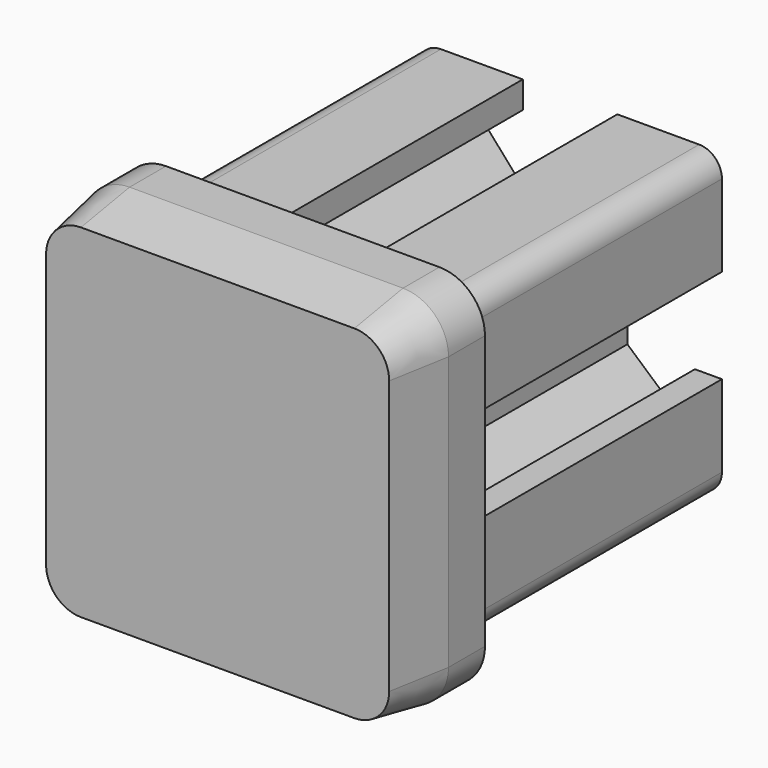
from build123d import *

# Parameters (mm, degrees)
F1_DEPTH = 25
F2_R     = 1.5
F4_DEPTH = 4
F4_TAPER = 10
F5_DEPTH = 3


with BuildPart() as f1:
    # F0 (on Front) → F1 (new body)
    with BuildSketch(Plane.XZ):
        Polygon((10, 3.1115), (10, 10), (3.1115, 10), (3.1115, 8.222), (5.461, 8.222), (5.461, 6.444), (3.1115, 3.777), (0, 3.777), (-3.1115, 3.777), (-5.461, 6.444), (-5.461, 8.222), (-3.1115, 8.222), (-3.1115, 10), (-10, 10), (-10, 3.1115), (-8.222, 3.1115), (-8.222, 5.461), (-6.444, 5.461), (-3.777, 3.1115), (-3.777, 0), (-3.777, -3.1115), (-6.444, -5.461), (-8.222, -5.461), (-8.222, -3.1115), (-10, -3.1115), (-10, -10), (-3.1115, -10), (-3.1115, -8.222), (-5.461, -8.222), (-5.461, -6.444), (-3.1115, -3.777), (0, -3.777), (3.1115, -3.777), (5.461, -6.444), (5.461, -8.222), (3.1115, -8.222), (3.1115, -10), (10, -10), (10, -3.1115), (8.222, -3.1115), (8.222, -5.461), (6.444, -5.461), (3.777, -3.1115), (3.777, 0), (3.777, 3.1115), (6.444, 5.461), (8.222, 5.461), (8.222, 3.1115), align=None)
    extrude(amount=F1_DEPTH)

    # F2
    f2_edges = [f1.edges().sort_by_distance(p)[0] for p in [
        (-10, -12.5, 10),
        (10, -12.5, 10),
        (10, -12.5, -10),
        (-10, -12.5, -10),
    ]]
    fillet(f2_edges, radius=F2_R)


with BuildPart() as f4:
    # F3 (on face) → F4 (new body)
    with BuildSketch(Plane.XZ.offset(25)):
        with BuildLine():
            Line((9, 12), (-9, 12))
            ThreePointArc((-9, 12), (-11.1213203436, 11.1213203436), (-12, 9))
            Line((-12, 9), (-12, -9))
            ThreePointArc((-12, -9), (-11.1213203436, -11.1213203436), (-9, -12))
            Line((-9, -12), (9, -12))
            ThreePointArc((9, -12), (11.1213203436, -11.1213203436), (12, -9))
            Line((12, -9), (12, 9))
            ThreePointArc((12, 9), (11.1213203436, 11.1213203436), (9, 12))
        make_face()
        with BuildLine():
            Line((10, 8.5), (10, 3.1115))
            Line((10, 3.1115), (8.222, 3.1115))
            Line((8.222, 3.1115), (8.222, 5.461))
            Line((8.222, 5.461), (6.444, 5.461))
            Line((6.444, 5.461), (3.777, 3.1115))
            Line((3.777, 3.1115), (3.777, -3.1115))
            Line((3.777, -3.1115), (6.444, -5.461))
            Line((6.444, -5.461), (8.222, -5.461))
            Line((8.222, -5.461), (8.222, -3.1115))
            Line((8.222, -3.1115), (10, -3.1115))
            Line((10, -3.1115), (10, -8.5))
            ThreePointArc((10, -8.5), (9.5606601718, -9.5606601718), (8.5, -10))
            Line((8.5, -10), (3.1115, -10))
            Line((3.1115, -10), (3.1115, -8.222))
            Line((3.1115, -8.222), (5.461, -8.222))
            Line((5.461, -8.222), (5.461, -6.444))
            Line((5.461, -6.444), (3.1115, -3.777))
            Line((3.1115, -3.777), (-3.1115, -3.777))
            Line((-3.1115, -3.777), (-5.461, -6.444))
            Line((-5.461, -6.444), (-5.461, -8.222))
            Line((-5.461, -8.222), (-3.1115, -8.222))
            Line((-3.1115, -8.222), (-3.1115, -10))
            Line((-3.1115, -10), (-8.5, -10))
            ThreePointArc((-8.5, -10), (-9.5606601718, -9.5606601718), (-10, -8.5))
            Line((-10, -8.5), (-10, -3.1115))
            Line((-10, -3.1115), (-8.222, -3.1115))
            Line((-8.222, -3.1115), (-8.222, -5.461))
            Line((-8.222, -5.461), (-6.444, -5.461))
            Line((-6.444, -5.461), (-3.777, -3.1115))
            Line((-3.777, -3.1115), (-3.777, 3.1115))
            Line((-3.777, 3.1115), (-6.444, 5.461))
            Line((-6.444, 5.461), (-8.222, 5.461))
            Line((-8.222, 5.461), (-8.222, 3.1115))
            Line((-8.222, 3.1115), (-10, 3.1115))
            Line((-10, 3.1115), (-10, 8.5))
            ThreePointArc((-10, 8.5), (-9.5606601718, 9.5606601718), (-8.5, 10))
            Line((-8.5, 10), (-3.1115, 10))
            Line((-3.1115, 10), (-3.1115, 8.222))
            Line((-3.1115, 8.222), (-5.461, 8.222))
            Line((-5.461, 8.222), (-5.461, 6.444))
            Line((-5.461, 6.444), (-3.1115, 3.777))
            Line((-3.1115, 3.777), (3.1115, 3.777))
            Line((3.1115, 3.777), (5.461, 6.444))
            Line((5.461, 6.444), (5.461, 8.222))
            Line((5.461, 8.222), (3.1115, 8.222))
            Line((3.1115, 8.222), (3.1115, 10))
            Line((3.1115, 10), (8.5, 10))
            ThreePointArc((8.5, 10), (9.5606601718, 9.5606601718), (10, 8.5))
        make_face(mode=Mode.SUBTRACT)
        with BuildLine():
            Line((8.222, 3.1115), (10, 3.1115))
            Line((10, 3.1115), (10, 8.5))
            ThreePointArc((10, 8.5), (9.5606601718, 9.5606601718), (8.5, 10))
            Line((8.5, 10), (3.1115, 10))
            Line((3.1115, 10), (3.1115, 8.222))
            Line((3.1115, 8.222), (5.461, 8.222))
            Line((5.461, 8.222), (5.461, 6.444))
            Line((5.461, 6.444), (3.1115, 3.777))
            Line((3.1115, 3.777), (-3.1115, 3.777))
            Line((-3.1115, 3.777), (-5.461, 6.444))
            Line((-5.461, 6.444), (-5.461, 8.222))
            Line((-5.461, 8.222), (-3.1115, 8.222))
            Line((-3.1115, 8.222), (-3.1115, 10))
            Line((-3.1115, 10), (-8.5, 10))
            ThreePointArc((-8.5, 10), (-9.5606601718, 9.5606601718), (-10, 8.5))
            Line((-10, 8.5), (-10, 3.1115))
            Line((-10, 3.1115), (-8.222, 3.1115))
            Line((-8.222, 3.1115), (-8.222, 5.461))
            Line((-8.222, 5.461), (-6.444, 5.461))
            Line((-6.444, 5.461), (-3.777, 3.1115))
            Line((-3.777, 3.1115), (-3.777, -3.1115))
            Line((-3.777, -3.1115), (-6.444, -5.461))
            Line((-6.444, -5.461), (-8.222, -5.461))
            Line((-8.222, -5.461), (-8.222, -3.1115))
            Line((-8.222, -3.1115), (-10, -3.1115))
            Line((-10, -3.1115), (-10, -8.5))
            ThreePointArc((-10, -8.5), (-9.5606601718, -9.5606601718), (-8.5, -10))
            Line((-8.5, -10), (-3.1115, -10))
            Line((-3.1115, -10), (-3.1115, -8.222))
            Line((-3.1115, -8.222), (-5.461, -8.222))
            Line((-5.461, -8.222), (-5.461, -6.444))
            Line((-5.461, -6.444), (-3.1115, -3.777))
            Line((-3.1115, -3.777), (3.1115, -3.777))
            Line((3.1115, -3.777), (5.461, -6.444))
            Line((5.461, -6.444), (5.461, -8.222))
            Line((5.461, -8.222), (3.1115, -8.222))
            Line((3.1115, -8.222), (3.1115, -10))
            Line((3.1115, -10), (8.5, -10))
            ThreePointArc((8.5, -10), (9.5606601718, -9.5606601718), (10, -8.5))
            Line((10, -8.5), (10, -3.1115))
            Line((10, -3.1115), (8.222, -3.1115))
            Line((8.222, -3.1115), (8.222, -5.461))
            Line((8.222, -5.461), (6.444, -5.461))
            Line((6.444, -5.461), (3.777, -3.1115))
            Line((3.777, -3.1115), (3.777, 3.1115))
            Line((3.777, 3.1115), (6.444, 5.461))
            Line((6.444, 5.461), (8.222, 5.461))
            Line((8.222, 5.461), (8.222, 3.1115))
        make_face()
    extrude(amount=F4_DEPTH, taper=F4_TAPER)

    # F3 (on face) → F5 (join)
    with BuildSketch(Plane.XZ.offset(25)):
        with BuildLine():
            Line((9, 12), (-9, 12))
            ThreePointArc((-9, 12), (-11.1213203436, 11.1213203436), (-12, 9))
            Line((-12, 9), (-12, -9))
            ThreePointArc((-12, -9), (-11.1213203436, -11.1213203436), (-9, -12))
            Line((-9, -12), (9, -12))
            ThreePointArc((9, -12), (11.1213203436, -11.1213203436), (12, -9))
            Line((12, -9), (12, 9))
            ThreePointArc((12, 9), (11.1213203436, 11.1213203436), (9, 12))
        make_face()
        with BuildLine():
            Line((10, 8.5), (10, 3.1115))
            Line((10, 3.1115), (8.222, 3.1115))
            Line((8.222, 3.1115), (8.222, 5.461))
            Line((8.222, 5.461), (6.444, 5.461))
            Line((6.444, 5.461), (3.777, 3.1115))
            Line((3.777, 3.1115), (3.777, -3.1115))
            Line((3.777, -3.1115), (6.444, -5.461))
            Line((6.444, -5.461), (8.222, -5.461))
            Line((8.222, -5.461), (8.222, -3.1115))
            Line((8.222, -3.1115), (10, -3.1115))
            Line((10, -3.1115), (10, -8.5))
            ThreePointArc((10, -8.5), (9.5606601718, -9.5606601718), (8.5, -10))
            Line((8.5, -10), (3.1115, -10))
            Line((3.1115, -10), (3.1115, -8.222))
            Line((3.1115, -8.222), (5.461, -8.222))
            Line((5.461, -8.222), (5.461, -6.444))
            Line((5.461, -6.444), (3.1115, -3.777))
            Line((3.1115, -3.777), (-3.1115, -3.777))
            Line((-3.1115, -3.777), (-5.461, -6.444))
            Line((-5.461, -6.444), (-5.461, -8.222))
            Line((-5.461, -8.222), (-3.1115, -8.222))
            Line((-3.1115, -8.222), (-3.1115, -10))
            Line((-3.1115, -10), (-8.5, -10))
            ThreePointArc((-8.5, -10), (-9.5606601718, -9.5606601718), (-10, -8.5))
            Line((-10, -8.5), (-10, -3.1115))
            Line((-10, -3.1115), (-8.222, -3.1115))
            Line((-8.222, -3.1115), (-8.222, -5.461))
            Line((-8.222, -5.461), (-6.444, -5.461))
            Line((-6.444, -5.461), (-3.777, -3.1115))
            Line((-3.777, -3.1115), (-3.777, 3.1115))
            Line((-3.777, 3.1115), (-6.444, 5.461))
            Line((-6.444, 5.461), (-8.222, 5.461))
            Line((-8.222, 5.461), (-8.222, 3.1115))
            Line((-8.222, 3.1115), (-10, 3.1115))
            Line((-10, 3.1115), (-10, 8.5))
            ThreePointArc((-10, 8.5), (-9.5606601718, 9.5606601718), (-8.5, 10))
            Line((-8.5, 10), (-3.1115, 10))
            Line((-3.1115, 10), (-3.1115, 8.222))
            Line((-3.1115, 8.222), (-5.461, 8.222))
            Line((-5.461, 8.222), (-5.461, 6.444))
            Line((-5.461, 6.444), (-3.1115, 3.777))
            Line((-3.1115, 3.777), (3.1115, 3.777))
            Line((3.1115, 3.777), (5.461, 6.444))
            Line((5.461, 6.444), (5.461, 8.222))
            Line((5.461, 8.222), (3.1115, 8.222))
            Line((3.1115, 8.222), (3.1115, 10))
            Line((3.1115, 10), (8.5, 10))
            ThreePointArc((8.5, 10), (9.5606601718, 9.5606601718), (10, 8.5))
        make_face(mode=Mode.SUBTRACT)
    extrude(amount=-F5_DEPTH)


solid = Compound([f1.part, f4.part])
